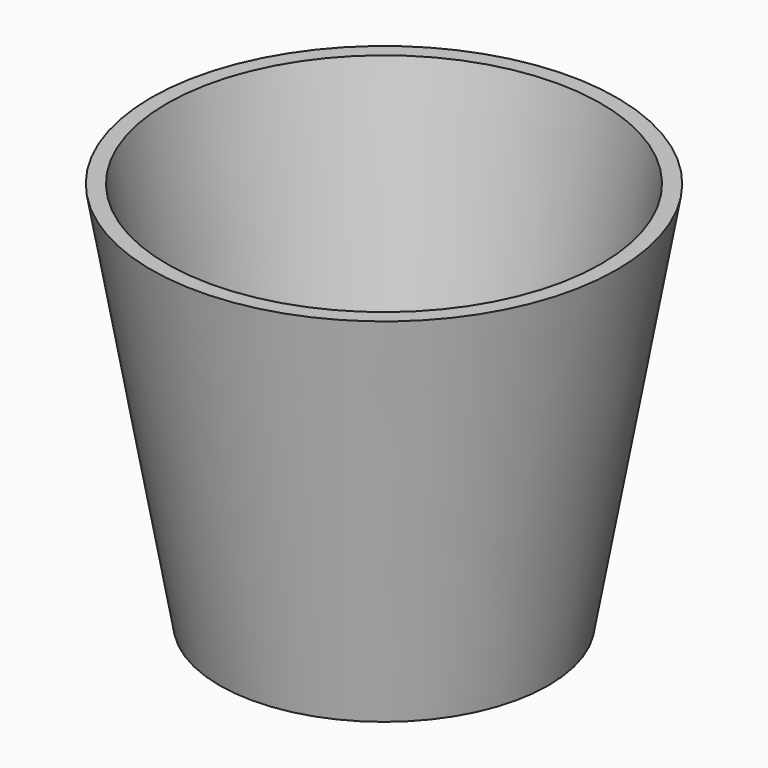
from build123d import *

# Parameters (mm, degrees)
F3_T     = -2.54
F5_D     = 7.62
F5_DEPTH = 38.101


# Not quite as in the source:
# - a feature of the source that left no trace in its solid (it failed there, or was rolled back) is left out


with BuildPart() as f1:
    # F0 (on Front) → F1 (revolve)
    with BuildSketch(Plane.XZ):
        Polygon((0, 0), (0, 63.5), (-38.1, 63.5), (-26.903236725, 0), align=None)
    revolve(axis=Axis((0, 0, 31.75), (0, 0, 1)))

    # F3
    f3_openings = [f1.faces().sort_by_distance(p)[0] for p in [
        (0, 0, 63.5),
    ]]
    offset(amount=F3_T, openings=f3_openings)

    # F5 (through all, one way)
    with BuildSketch(Plane.YZ):
        with Locations((0, 12.7)):
            Circle(F5_D / 2)
    extrude(amount=-F5_DEPTH, mode=Mode.SUBTRACT)


solid = f1.part
